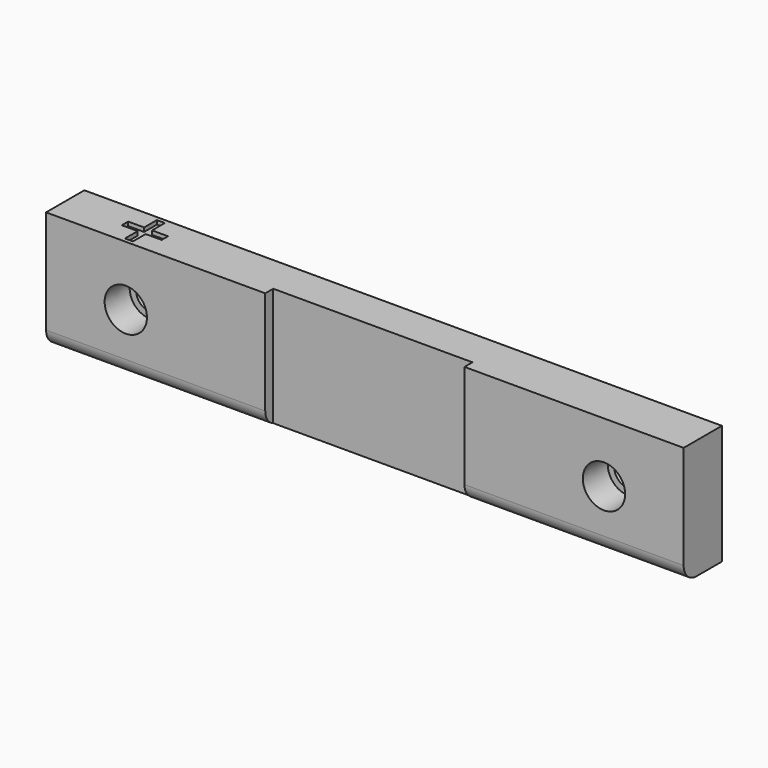
from build123d import *

# Parameters (mm, degrees)
F1_DEPTH  = 15
F4_R      = 2.55
F2_R      = 2.655
F7_D      = 3.5
F8_F1_R   = 2
F9_W      = 2
F9_H      = 1
F9_W_2    = 1
F9_H_2    = 2
F10_DEPTH = 0.5


with BuildPart() as f1:
    # F0 (on Top) → F1 (new body)
    with BuildSketch(Plane.XY):
        Polygon((12.5, -3), (40, -3), (40, 3), (-40, 3), (-40, -3), (-12.5, -3), (-12.5, -1.75), (12.5, -1.75), align=None)
    extrude(amount=F1_DEPTH)

    # F4 (on offset) → F5 section 0
    with BuildSketch(Plane.XZ.offset(-0.8)):
        with Locations((-30, 7.5)):
            Circle(F4_R)
    # F2 (on face) → F5 section 1
    with BuildSketch(Plane.XZ.offset(3)):
        with Locations((-30, 7.5)):
            Circle(F2_R)
    loft(mode=Mode.SUBTRACT)

    # F2 (on face) → F6 section 0
    with BuildSketch(Plane.XZ.offset(3)):
        with Locations((30, 7.5)):
            Circle(F2_R)
    # F4 (on offset) → F6 section 1
    with BuildSketch(Plane.XZ.offset(-0.8)):
        with Locations((30, 7.5)):
            Circle(F4_R)
    loft(mode=Mode.SUBTRACT)

    # F7 (through all)
    with Locations(Plane.XZ.offset(-0.8)):
        with Locations((30, 7.5), (-30, 7.5)):
            Hole(F7_D / 2)

    # F8: fillet of radius 2 on 2 edges, made by hand

    # F8_f1
    f8_f1_edges = [f1.edges().sort_by_distance(p)[0] for p in [
        (26.25, -3, 0),
    ]]
    fillet(f8_f1_edges, radius=F8_F1_R)

    # F9 (on face) → F10 (cut)
    with BuildSketch(Plane.XY.offset(15)):
        with Locations((-31.5, 0)):
            Rectangle(F9_W, F9_H)
        with Locations((-30, 0)):
            Rectangle(F9_W_2, F9_H)
        with Locations((-28.5, 0)):
            Rectangle(F9_W, F9_H)
        with Locations((-30, 1.5)):
            Rectangle(F9_W_2, F9_H_2)
        with Locations((-30, -1.5)):
            Rectangle(F9_W_2, F9_H_2)
    extrude(amount=-F10_DEPTH, mode=Mode.SUBTRACT)


solid = f1.part
